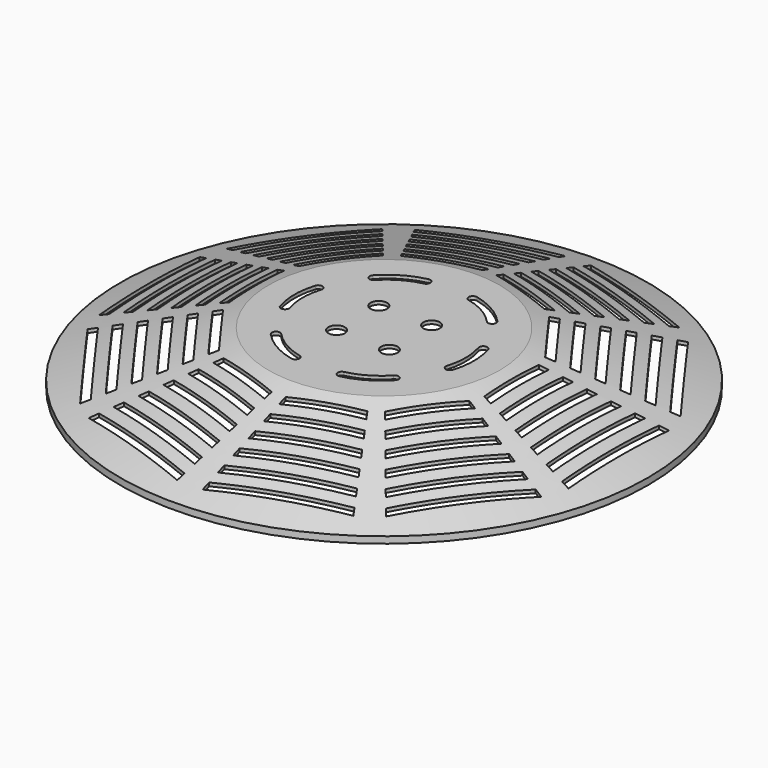
from build123d import *

# Parameters (mm, degrees)
F2_T      = -1.27
F4_DEPTH  = 20.321
F5_COUNT  = 6
F8_DEPTH  = 25.4
F9_COUNT  = 10
F11_R     = 3.175
F12_DEPTH = 20.321


# Not quite as in the source:
# - a feature of the source that left no trace in its solid (it failed there, or was rolled back) is left out


with BuildPart() as f1:
    # F0 (on Front) → F1 (revolve)
    with BuildSketch(Plane.XZ):
        Polygon((0, 20.32), (0, 0), (101.6, 0), (101.6, 2.54), (44.45, 20.32), align=None)
    revolve(axis=Axis((0, 0, 10.16), (0, 0, 1)))

    # F2
    f2_openings = [f1.faces().sort_by_distance(p)[0] for p in [
        (0, 0, 0),
    ]]
    offset(amount=F2_T, openings=f2_openings)


with BuildPart() as f4:
    # F3 (on face) → F4 (new body, through all)
    with BuildSketch(Plane.XY.offset(20.32)):
        with BuildLine():
            ThreePointArc((-30.2338708511, -7.5303529412), (-31.3758044694, 0), (-30.2338708511, 7.5303529412))
            ThreePointArc((-30.2338708511, 7.5303529412), (-31.2793529412, 9.5171291489), (-33.2661291489, 8.4716470588))
            ThreePointArc((-33.2661291489, 8.4716470588), (-34.5508044694, 0), (-33.2661291489, -8.4716470588))
            ThreePointArc((-33.2661291489, -8.4716470588), (-31.2793529412, -9.5171291489), (-30.2338708511, -7.5303529412))
        make_face()
    extrude(amount=-F4_DEPTH)


with BuildPart() as f5_1:
    # F5: instance of F4
    add(f4.part.rotate(Axis((0, 0, 2.54), (0, 0, 1)), 1 * 360 / F5_COUNT))


with BuildPart() as f5_2:
    # F5: instance of F4
    add(f4.part.rotate(Axis((0, 0, 2.54), (0, 0, 1)), 2 * 360 / F5_COUNT))


with BuildPart() as f5_3:
    # F5: instance of F4
    add(f4.part.rotate(Axis((0, 0, 2.54), (0, 0, 1)), 3 * 360 / F5_COUNT))


with BuildPart() as f5_4:
    # F5: instance of F4
    add(f4.part.rotate(Axis((0, 0, 2.54), (0, 0, 1)), 4 * 360 / F5_COUNT))


with BuildPart() as f5_5:
    # F5: instance of F4
    add(f4.part.rotate(Axis((0, 0, 2.54), (0, 0, 1)), 5 * 360 / F5_COUNT))


with BuildPart() as f1_1:
    add(f1.part)

    # F6: cut F4, F5_1, F5_2, F5_3, F5_4, F5_5
    add(f4.part, mode=Mode.SUBTRACT)
    add(f5_1.part, mode=Mode.SUBTRACT)
    add(f5_2.part, mode=Mode.SUBTRACT)
    add(f5_3.part, mode=Mode.SUBTRACT)
    add(f5_4.part, mode=Mode.SUBTRACT)
    add(f5_5.part, mode=Mode.SUBTRACT)


with BuildPart() as f8:
    # F7 (on face) → F8 (new body)
    with BuildSketch(Plane.XY.offset(20.32)):
        Polygon((-79.5490319755, -21.3150988765), (-79.5490319755, 21.3150988765), (-82.7240319755, 22.1658375625), (-82.7240319755, -22.1658375625), align=None)
    extrude(amount=-F8_DEPTH)


with BuildPart() as f8b:
    # F7 (on face) → F8, piece 2 (new body)
    with BuildSketch(Plane.XY.offset(20.32)):
        Polygon((-71.9290319755, -19.2733260302), (-71.9290319755, 19.2733260302), (-75.1040319755, 20.1240647162), (-75.1040319755, -20.1240647162), align=None)
    extrude(amount=-F8_DEPTH)


with BuildPart() as f8c:
    # F7 (on face) → F8, piece 3 (new body)
    with BuildSketch(Plane.XY.offset(20.32)):
        Polygon((-64.3090319755, -17.2315531839), (-64.3090319755, 17.2315531839), (-67.4840319755, 18.0822918698), (-67.4840319755, -18.0822918698), align=None)
    extrude(amount=-F8_DEPTH)


with BuildPart() as f8d:
    # F7 (on face) → F8, piece 4 (new body)
    with BuildSketch(Plane.XY.offset(20.32)):
        Polygon((-56.6890319755, -15.1897803375), (-56.6890319755, 15.1897803375), (-59.8640319755, 16.0405190235), (-59.8640319755, -16.0405190235), align=None)
    extrude(amount=-F8_DEPTH)


with BuildPart() as f8e:
    # F7 (on face) → F8, piece 5 (new body)
    with BuildSketch(Plane.XY.offset(20.32)):
        Polygon((-49.0690319755, -13.1480074912), (-49.0690319755, 13.1480074912), (-52.2440319755, 13.9987461772), (-52.2440319755, -13.9987461772), align=None)
    extrude(amount=-F8_DEPTH)


with BuildPart() as f8f:
    # F7 (on face) → F8, piece 6 (new body)
    with BuildSketch(Plane.XY.offset(20.32)):
        Polygon((-87.1690319755, -23.3568717228), (-87.1690319755, 23.3568717228), (-90.3440319755, 24.2076104088), (-90.3440319755, -24.2076104088), align=None)
    extrude(amount=-F8_DEPTH)


with BuildPart() as f9_1:
    # F9: instance of F8f
    add(f8f.part.rotate(Axis((0, 0, 2.54), (0, 0, 1)), 1 * 360 / F9_COUNT))


with BuildPart() as f9_2:
    # F9: instance of F8f
    add(f8f.part.rotate(Axis((0, 0, 2.54), (0, 0, 1)), 2 * 360 / F9_COUNT))


with BuildPart() as f9_3:
    # F9: instance of F8f
    add(f8f.part.rotate(Axis((0, 0, 2.54), (0, 0, 1)), 3 * 360 / F9_COUNT))


with BuildPart() as f9_4:
    # F9: instance of F8f
    add(f8f.part.rotate(Axis((0, 0, 2.54), (0, 0, 1)), 4 * 360 / F9_COUNT))


with BuildPart() as f9_5:
    # F9: instance of F8f
    add(f8f.part.rotate(Axis((0, 0, 2.54), (0, 0, 1)), 5 * 360 / F9_COUNT))


with BuildPart() as f9_6:
    # F9: instance of F8f
    add(f8f.part.rotate(Axis((0, 0, 2.54), (0, 0, 1)), 6 * 360 / F9_COUNT))


with BuildPart() as f9_7:
    # F9: instance of F8f
    add(f8f.part.rotate(Axis((0, 0, 2.54), (0, 0, 1)), 7 * 360 / F9_COUNT))


with BuildPart() as f9_8:
    # F9: instance of F8f
    add(f8f.part.rotate(Axis((0, 0, 2.54), (0, 0, 1)), 8 * 360 / F9_COUNT))


with BuildPart() as f9_9:
    # F9: instance of F8f
    add(f8f.part.rotate(Axis((0, 0, 2.54), (0, 0, 1)), 9 * 360 / F9_COUNT))


with BuildPart() as f9_10:
    # F9: instance of F8
    add(f8.part.rotate(Axis((0, 0, 2.54), (0, 0, 1)), 1 * 360 / F9_COUNT))


with BuildPart() as f9_11:
    # F9: instance of F8
    add(f8.part.rotate(Axis((0, 0, 2.54), (0, 0, 1)), 2 * 360 / F9_COUNT))


with BuildPart() as f9_12:
    # F9: instance of F8
    add(f8.part.rotate(Axis((0, 0, 2.54), (0, 0, 1)), 3 * 360 / F9_COUNT))


with BuildPart() as f9_13:
    # F9: instance of F8
    add(f8.part.rotate(Axis((0, 0, 2.54), (0, 0, 1)), 4 * 360 / F9_COUNT))


with BuildPart() as f9_14:
    # F9: instance of F8
    add(f8.part.rotate(Axis((0, 0, 2.54), (0, 0, 1)), 5 * 360 / F9_COUNT))


with BuildPart() as f9_15:
    # F9: instance of F8
    add(f8.part.rotate(Axis((0, 0, 2.54), (0, 0, 1)), 6 * 360 / F9_COUNT))


with BuildPart() as f9_16:
    # F9: instance of F8
    add(f8.part.rotate(Axis((0, 0, 2.54), (0, 0, 1)), 7 * 360 / F9_COUNT))


with BuildPart() as f9_17:
    # F9: instance of F8
    add(f8.part.rotate(Axis((0, 0, 2.54), (0, 0, 1)), 8 * 360 / F9_COUNT))


with BuildPart() as f9_18:
    # F9: instance of F8
    add(f8.part.rotate(Axis((0, 0, 2.54), (0, 0, 1)), 9 * 360 / F9_COUNT))


with BuildPart() as f9_19:
    # F9: instance of F8b
    add(f8b.part.rotate(Axis((0, 0, 2.54), (0, 0, 1)), 1 * 360 / F9_COUNT))


with BuildPart() as f9_20:
    # F9: instance of F8b
    add(f8b.part.rotate(Axis((0, 0, 2.54), (0, 0, 1)), 2 * 360 / F9_COUNT))


with BuildPart() as f9_21:
    # F9: instance of F8b
    add(f8b.part.rotate(Axis((0, 0, 2.54), (0, 0, 1)), 3 * 360 / F9_COUNT))


with BuildPart() as f9_22:
    # F9: instance of F8b
    add(f8b.part.rotate(Axis((0, 0, 2.54), (0, 0, 1)), 4 * 360 / F9_COUNT))


with BuildPart() as f9_23:
    # F9: instance of F8b
    add(f8b.part.rotate(Axis((0, 0, 2.54), (0, 0, 1)), 5 * 360 / F9_COUNT))


with BuildPart() as f9_24:
    # F9: instance of F8b
    add(f8b.part.rotate(Axis((0, 0, 2.54), (0, 0, 1)), 6 * 360 / F9_COUNT))


with BuildPart() as f9_25:
    # F9: instance of F8b
    add(f8b.part.rotate(Axis((0, 0, 2.54), (0, 0, 1)), 7 * 360 / F9_COUNT))


with BuildPart() as f9_26:
    # F9: instance of F8b
    add(f8b.part.rotate(Axis((0, 0, 2.54), (0, 0, 1)), 8 * 360 / F9_COUNT))


with BuildPart() as f9_27:
    # F9: instance of F8b
    add(f8b.part.rotate(Axis((0, 0, 2.54), (0, 0, 1)), 9 * 360 / F9_COUNT))


with BuildPart() as f9_28:
    # F9: instance of F8c
    add(f8c.part.rotate(Axis((0, 0, 2.54), (0, 0, 1)), 1 * 360 / F9_COUNT))


with BuildPart() as f9_29:
    # F9: instance of F8c
    add(f8c.part.rotate(Axis((0, 0, 2.54), (0, 0, 1)), 2 * 360 / F9_COUNT))


with BuildPart() as f9_30:
    # F9: instance of F8c
    add(f8c.part.rotate(Axis((0, 0, 2.54), (0, 0, 1)), 3 * 360 / F9_COUNT))


with BuildPart() as f9_31:
    # F9: instance of F8c
    add(f8c.part.rotate(Axis((0, 0, 2.54), (0, 0, 1)), 4 * 360 / F9_COUNT))


with BuildPart() as f9_32:
    # F9: instance of F8c
    add(f8c.part.rotate(Axis((0, 0, 2.54), (0, 0, 1)), 5 * 360 / F9_COUNT))


with BuildPart() as f9_33:
    # F9: instance of F8c
    add(f8c.part.rotate(Axis((0, 0, 2.54), (0, 0, 1)), 6 * 360 / F9_COUNT))


with BuildPart() as f9_34:
    # F9: instance of F8c
    add(f8c.part.rotate(Axis((0, 0, 2.54), (0, 0, 1)), 7 * 360 / F9_COUNT))


with BuildPart() as f9_35:
    # F9: instance of F8c
    add(f8c.part.rotate(Axis((0, 0, 2.54), (0, 0, 1)), 8 * 360 / F9_COUNT))


with BuildPart() as f9_36:
    # F9: instance of F8c
    add(f8c.part.rotate(Axis((0, 0, 2.54), (0, 0, 1)), 9 * 360 / F9_COUNT))


with BuildPart() as f9_37:
    # F9: instance of F8d
    add(f8d.part.rotate(Axis((0, 0, 2.54), (0, 0, 1)), 1 * 360 / F9_COUNT))


with BuildPart() as f9_38:
    # F9: instance of F8d
    add(f8d.part.rotate(Axis((0, 0, 2.54), (0, 0, 1)), 2 * 360 / F9_COUNT))


with BuildPart() as f9_39:
    # F9: instance of F8d
    add(f8d.part.rotate(Axis((0, 0, 2.54), (0, 0, 1)), 3 * 360 / F9_COUNT))


with BuildPart() as f9_40:
    # F9: instance of F8d
    add(f8d.part.rotate(Axis((0, 0, 2.54), (0, 0, 1)), 4 * 360 / F9_COUNT))


with BuildPart() as f9_41:
    # F9: instance of F8d
    add(f8d.part.rotate(Axis((0, 0, 2.54), (0, 0, 1)), 5 * 360 / F9_COUNT))


with BuildPart() as f9_42:
    # F9: instance of F8d
    add(f8d.part.rotate(Axis((0, 0, 2.54), (0, 0, 1)), 6 * 360 / F9_COUNT))


with BuildPart() as f9_43:
    # F9: instance of F8d
    add(f8d.part.rotate(Axis((0, 0, 2.54), (0, 0, 1)), 7 * 360 / F9_COUNT))


with BuildPart() as f9_44:
    # F9: instance of F8d
    add(f8d.part.rotate(Axis((0, 0, 2.54), (0, 0, 1)), 8 * 360 / F9_COUNT))


with BuildPart() as f9_45:
    # F9: instance of F8d
    add(f8d.part.rotate(Axis((0, 0, 2.54), (0, 0, 1)), 9 * 360 / F9_COUNT))


with BuildPart() as f9_46:
    # F9: instance of F8e
    add(f8e.part.rotate(Axis((0, 0, 2.54), (0, 0, 1)), 1 * 360 / F9_COUNT))


with BuildPart() as f9_47:
    # F9: instance of F8e
    add(f8e.part.rotate(Axis((0, 0, 2.54), (0, 0, 1)), 2 * 360 / F9_COUNT))


with BuildPart() as f9_48:
    # F9: instance of F8e
    add(f8e.part.rotate(Axis((0, 0, 2.54), (0, 0, 1)), 3 * 360 / F9_COUNT))


with BuildPart() as f9_49:
    # F9: instance of F8e
    add(f8e.part.rotate(Axis((0, 0, 2.54), (0, 0, 1)), 4 * 360 / F9_COUNT))


with BuildPart() as f9_50:
    # F9: instance of F8e
    add(f8e.part.rotate(Axis((0, 0, 2.54), (0, 0, 1)), 5 * 360 / F9_COUNT))


with BuildPart() as f9_51:
    # F9: instance of F8e
    add(f8e.part.rotate(Axis((0, 0, 2.54), (0, 0, 1)), 6 * 360 / F9_COUNT))


with BuildPart() as f9_52:
    # F9: instance of F8e
    add(f8e.part.rotate(Axis((0, 0, 2.54), (0, 0, 1)), 7 * 360 / F9_COUNT))


with BuildPart() as f9_53:
    # F9: instance of F8e
    add(f8e.part.rotate(Axis((0, 0, 2.54), (0, 0, 1)), 8 * 360 / F9_COUNT))


with BuildPart() as f9_54:
    # F9: instance of F8e
    add(f8e.part.rotate(Axis((0, 0, 2.54), (0, 0, 1)), 9 * 360 / F9_COUNT))


with BuildPart() as f1_2:
    add(f1_1.part)

    # F10: cut F8f, F8e, F8d, F8c, F8b, F8, F9_1, F9_46, F9_37, F9_28, F9_19, F9_10, F9_2, F9_47, F9_38, F9_29, F9_20, F9_11, F9_3, F9_48, F9_39, F9_30, F9_21, F9_12, F9_4, F9_49, F9_40, F9_31, F9_22, F9_13, F9_5, F9_50, F9_41, F9_32, F9_23, F9_14, F9_6, F9_51, F9_42, F9_33, F9_24, F9_15, F9_7, F9_52, F9_43, F9_34, F9_25, F9_16, F9_8, F9_53, F9_44, F9_35, F9_26, F9_17, F9_9, F9_54, F9_45, F9_36, F9_27, F9_18
    add(f8f.part, mode=Mode.SUBTRACT)
    add(f8e.part, mode=Mode.SUBTRACT)
    add(f8d.part, mode=Mode.SUBTRACT)
    add(f8c.part, mode=Mode.SUBTRACT)
    add(f8b.part, mode=Mode.SUBTRACT)
    add(f8.part, mode=Mode.SUBTRACT)
    add(f9_1.part, mode=Mode.SUBTRACT)
    add(f9_46.part, mode=Mode.SUBTRACT)
    add(f9_37.part, mode=Mode.SUBTRACT)
    add(f9_28.part, mode=Mode.SUBTRACT)
    add(f9_19.part, mode=Mode.SUBTRACT)
    add(f9_10.part, mode=Mode.SUBTRACT)
    add(f9_2.part, mode=Mode.SUBTRACT)
    add(f9_47.part, mode=Mode.SUBTRACT)
    add(f9_38.part, mode=Mode.SUBTRACT)
    add(f9_29.part, mode=Mode.SUBTRACT)
    add(f9_20.part, mode=Mode.SUBTRACT)
    add(f9_11.part, mode=Mode.SUBTRACT)
    add(f9_3.part, mode=Mode.SUBTRACT)
    add(f9_48.part, mode=Mode.SUBTRACT)
    add(f9_39.part, mode=Mode.SUBTRACT)
    add(f9_30.part, mode=Mode.SUBTRACT)
    add(f9_21.part, mode=Mode.SUBTRACT)
    add(f9_12.part, mode=Mode.SUBTRACT)
    add(f9_4.part, mode=Mode.SUBTRACT)
    add(f9_49.part, mode=Mode.SUBTRACT)
    add(f9_40.part, mode=Mode.SUBTRACT)
    add(f9_31.part, mode=Mode.SUBTRACT)
    add(f9_22.part, mode=Mode.SUBTRACT)
    add(f9_13.part, mode=Mode.SUBTRACT)
    add(f9_5.part, mode=Mode.SUBTRACT)
    add(f9_50.part, mode=Mode.SUBTRACT)
    add(f9_41.part, mode=Mode.SUBTRACT)
    add(f9_32.part, mode=Mode.SUBTRACT)
    add(f9_23.part, mode=Mode.SUBTRACT)
    add(f9_14.part, mode=Mode.SUBTRACT)
    add(f9_6.part, mode=Mode.SUBTRACT)
    add(f9_51.part, mode=Mode.SUBTRACT)
    add(f9_42.part, mode=Mode.SUBTRACT)
    add(f9_33.part, mode=Mode.SUBTRACT)
    add(f9_24.part, mode=Mode.SUBTRACT)
    add(f9_15.part, mode=Mode.SUBTRACT)
    add(f9_7.part, mode=Mode.SUBTRACT)
    add(f9_52.part, mode=Mode.SUBTRACT)
    add(f9_43.part, mode=Mode.SUBTRACT)
    add(f9_34.part, mode=Mode.SUBTRACT)
    add(f9_25.part, mode=Mode.SUBTRACT)
    add(f9_16.part, mode=Mode.SUBTRACT)
    add(f9_8.part, mode=Mode.SUBTRACT)
    add(f9_53.part, mode=Mode.SUBTRACT)
    add(f9_44.part, mode=Mode.SUBTRACT)
    add(f9_35.part, mode=Mode.SUBTRACT)
    add(f9_26.part, mode=Mode.SUBTRACT)
    add(f9_17.part, mode=Mode.SUBTRACT)
    add(f9_9.part, mode=Mode.SUBTRACT)
    add(f9_54.part, mode=Mode.SUBTRACT)
    add(f9_45.part, mode=Mode.SUBTRACT)
    add(f9_36.part, mode=Mode.SUBTRACT)
    add(f9_27.part, mode=Mode.SUBTRACT)
    add(f9_18.part, mode=Mode.SUBTRACT)

    # F11 (on face) → F12 (cut, through all)
    with BuildSketch(Plane.XY.offset(20.32)):
        with Locations((-10.16, -10.16)):
            Circle(F11_R)
        with Locations((-10.16, 10.16)):
            Circle(F11_R)
        with Locations((10.16, -10.16)):
            Circle(F11_R)
        with Locations((10.16, 10.16)):
            Circle(F11_R)
    extrude(amount=-F12_DEPTH, mode=Mode.SUBTRACT)


solid = f1_2.part
